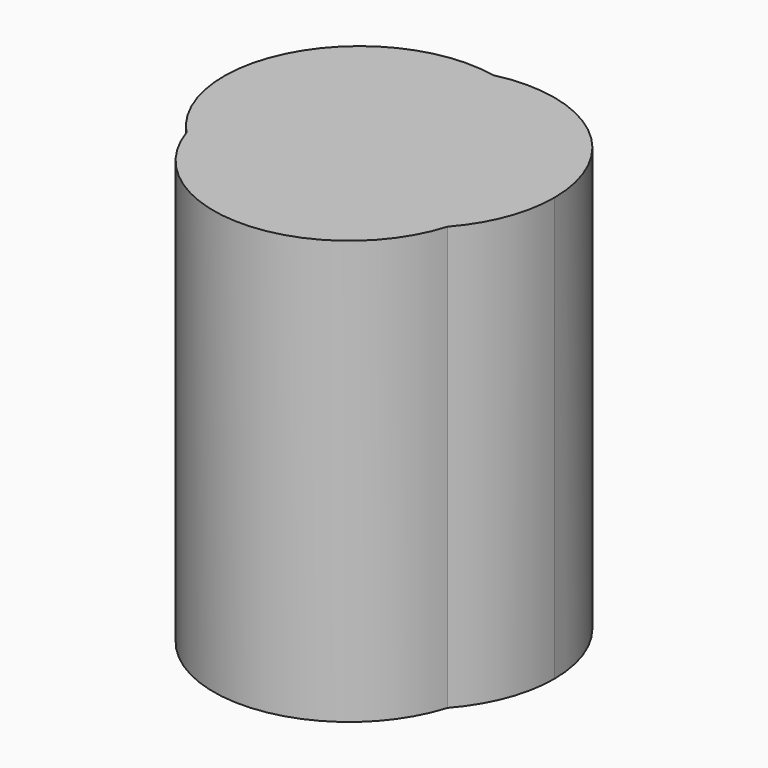
from build123d import *

# Parameters (mm, degrees)
F1_DEPTH = 5


with BuildPart() as f1:
    # F0 (on Top) → F1 (new body)
    with BuildSketch(Plane.XY):
        with BuildLine():
            ThreePointArc((0.0127623188, -1.3154877858), (0.9001120091, -0.7513032815), (1.2456412678, 0.2418246857))
            ThreePointArc((1.2456412678, 0.2418246857), (1.2253718915, 0.4956970091), (1.1650773221, 0.7431370404))
            ThreePointArc((1.1650773221, 0.7431370404), (-0.021224531, 1.2463674095), (-1.1937590183, 0.7118435401))
            ThreePointArc((-1.1937590183, 0.7118435401), (-1.0364939631, -0.5672465342), (0.0127623188, -1.3154877858))
        make_face()
        with BuildLine():
            ThreePointArc((1.1650773221, 0.7431370404), (1.2253718915, 0.4956970091), (1.2456412678, 0.2418246857))
            ThreePointArc((1.2456412678, 0.2418246857), (0.9001120091, -0.7513032815), (0.0127623188, -1.3154877858))
            ThreePointArc((0.0127623188, -1.3154877858), (0.8396230024, -1.2684634277), (1.5322002861, -0.8143196329))
            ThreePointArc((1.5322002861, -0.8143196329), (1.5829593264, -0.5863861437), (1.6, -0.3534918091))
            ThreePointArc((1.6, -0.3534918091), (1.4873001908, 0.2363710075), (1.1650773221, 0.7431370404))
        make_face()
        with BuildLine():
            ThreePointArc((-1.1937590183, 0.7118435401), (-0.021224531, 1.2463674095), (1.1650773221, 0.7431370404))
            ThreePointArc((1.1650773221, 0.7431370404), (0.7108972882, 1.4356544939), (-0.0286797832, 1.8083281878))
            ThreePointArc((-0.0286797832, 1.8083281878), (-0.7581101587, 1.4161659079), (-1.1937590183, 0.7118435401))
        make_face()
        with BuildLine():
            ThreePointArc((-0.0286797832, 1.8083281878), (0.7108972882, 1.4356544939), (1.1650773221, 0.7431370404))
            ThreePointArc((1.1650773221, 0.7431370404), (1.4873001908, 0.2363710075), (1.6, -0.3534918091))
            ThreePointArc((1.6, -0.3534918091), (1.5829593264, -0.5863861437), (1.5322002861, -0.8143196329))
            ThreePointArc((1.5322002861, -0.8143196329), (1.8334353195, -0.3190656686), (1.9384412678, 0.2510157163))
            ThreePointArc((1.9384412678, 0.2510157163), (1.331569235, 1.5054864576), (-0.0286797832, 1.8083281878))
        make_face()
        with BuildLine():
            ThreePointArc((1.5322002861, -0.8143196329), (0.8396230024, -1.2684634277), (0.0127623188, -1.3154877858))
            ThreePointArc((0.0127623188, -1.3154877858), (-0.8150548387, -1.2904152099), (-1.5194360543, -0.8548041638))
            ThreePointArc((-1.5194360543, -0.8548041638), (0.021224531, -1.9533510277), (1.5322002861, -0.8143196329))
        make_face()
        with BuildLine():
            ThreePointArc((-1.5194360543, -0.8548041638), (-0.8150548387, -1.2904152099), (0.0127623188, -1.3154877858))
            ThreePointArc((0.0127623188, -1.3154877858), (-1.0364939631, -0.5672465342), (-1.1937590183, 0.7118435401))
            ThreePointArc((-1.1937590183, 0.7118435401), (-1.5665098571, -0.0278434289), (-1.5194360543, -0.8548041638))
        make_face()
        with BuildLine():
            ThreePointArc((-1.1937590183, 0.7118435401), (-0.7581101587, 1.4161659079), (-0.0286797832, 1.8083281878))
            ThreePointArc((-0.0286797832, 1.8083281878), (-1.7505019511, 1.0233514685), (-1.5194360543, -0.8548041638))
            ThreePointArc((-1.5194360543, -0.8548041638), (-1.5665098571, -0.0278434289), (-1.1937590183, 0.7118435401))
        make_face()
    extrude(amount=F1_DEPTH)


solid = f1.part
